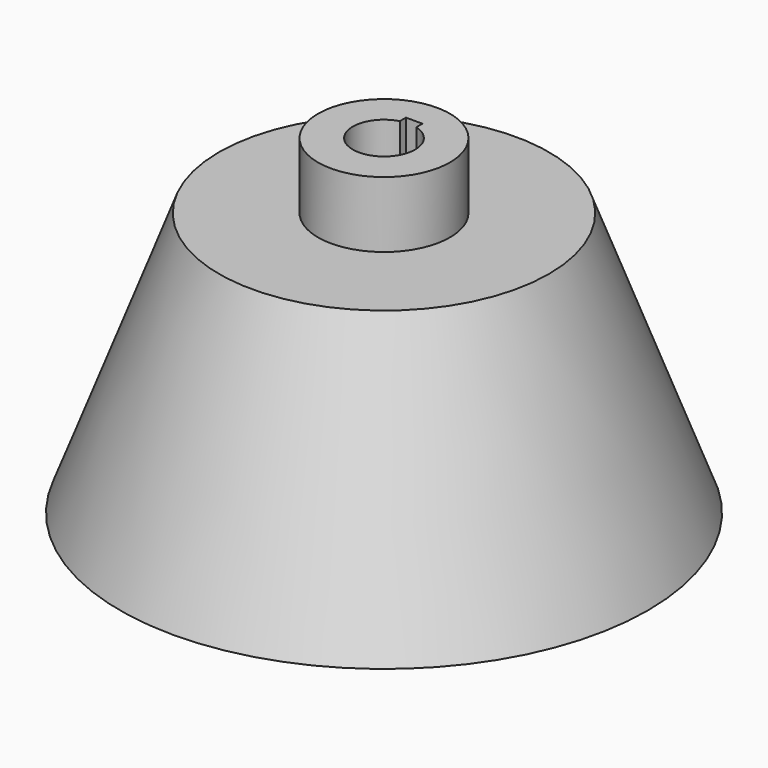
from build123d import *

# Parameters (mm, degrees)
F0_W            = 12.7
F0_H            = 12.7
F2_W            = 6
F2_H            = 25.4
F4_W            = 3.175
F4_H            = 7.2644
F5_DEPTH        = 63.501
F7_DEPTH        = 1.27
F7_COPIES_COUNT = 16


# Not quite as in the source:
# - a pattern or mirror of a feature is missing from the dataset's text; its kind, count and spacing are read off the source's solid


with BuildPart() as f1:
    # F0 (on Front) → F1 (revolve)
    with BuildSketch(Plane.XZ):
        Polygon((-50.8, 0), (0, 0), (0, 50.8), (-12.7, 50.8), (-31.75, 50.8), align=None)
        with Locations((-6.35, 57.15)):
            Rectangle(F0_W, F0_H)
    revolve(axis=Axis((0, 0, 25.4), (0, 0, 1)))

    # F2 (on Front) → F3 (revolve, cut)
    with BuildSketch(Plane.XZ):
        Polygon((-8.255, 38.1), (-38.1, 0), (0, 0), (0, 38.1), (-6, 38.1), align=None)
        with Locations((-3, 50.8)):
            Rectangle(F2_W, F2_H)
    revolve(axis=Axis((0, 0, 19.05), (0, 0, -1)), mode=Mode.SUBTRACT)

    # F4 (on Top) → F5 (cut, through all)
    with BuildSketch(Plane.XY):
        with Locations((0, 3.6322)):
            Rectangle(F4_W, F4_H)
    extrude(amount=F5_DEPTH, mode=Mode.SUBTRACT)

    # F6 (on Front) → F7 (cut, symmetric)
    with BuildSketch(Plane.XZ):
        Polygon((-12.7, 38.1), (-41.275, 0), (-34.925, 0), (-6.35, 38.1), align=None)
    f7 = extrude(amount=F7_DEPTH, both=True, mode=Mode.SUBTRACT)

    # F7_copies: F7 ×16 about axis
    f7_copies_axis = Axis((0, 0, 0), (0, 0, 1))
    for i in range(1, F7_COPIES_COUNT):
        add(f7.rotate(f7_copies_axis, i * 360 / F7_COPIES_COUNT), mode=Mode.SUBTRACT)


solid = f1.part
